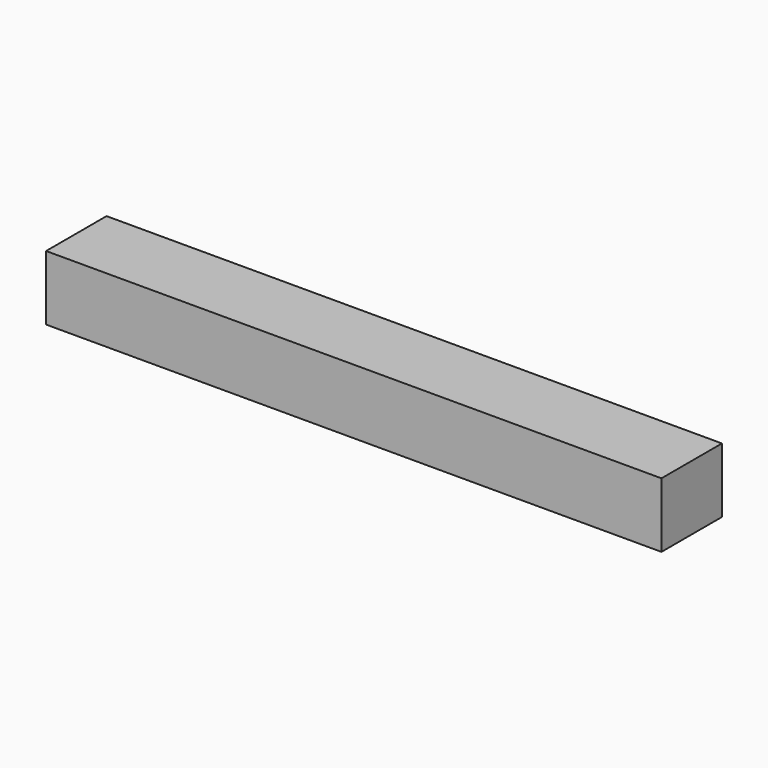
from build123d import *

# Parameters (mm, degrees)
F0_W     = 57
F0_H     = 6
F2_DEPTH = 7


# Not quite as in the source:
# - the program builds the solid bodies; features that only make, move or delete a surface that nothing else refers to are left out


with BuildPart() as f2:
    # F0 (on Front) → F2 (new body)
    with BuildSketch(Plane.XZ):
        with Locations((-0.8431142196, -23.1101376831)):
            Rectangle(F0_W, F0_H)
    extrude(amount=F2_DEPTH)


solid = f2.part
